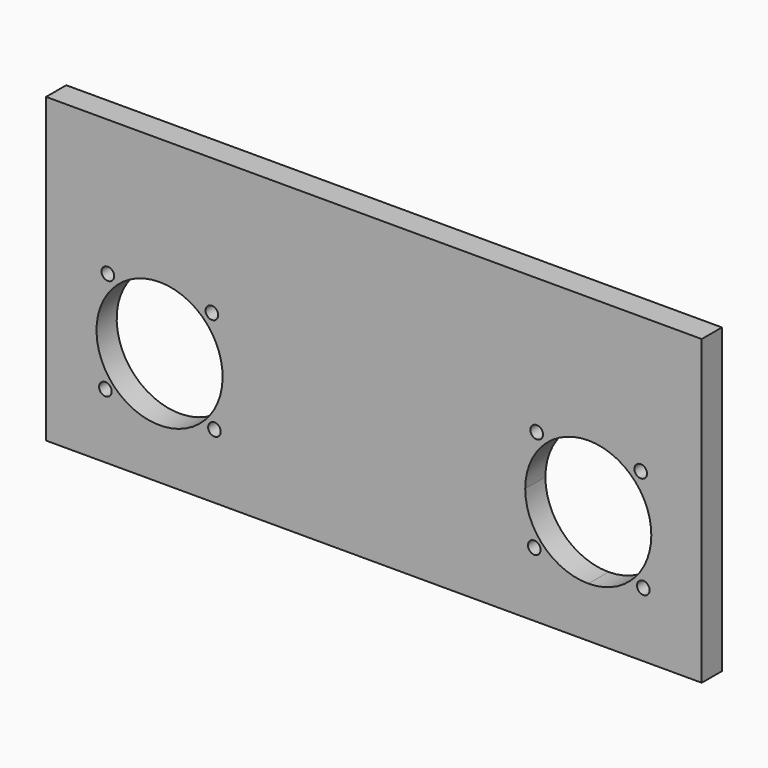
from build123d import *

# Parameters (mm, degrees)
F0_W     = 330.2
F0_H     = 152.4
F1_DEPTH = 12.7
F2_R     = 3.175
F3_DEPTH = 25.4


with BuildPart() as f1:
    # F0 (on Front) → F1 (new body)
    with BuildSketch(Plane.XZ):
        with Locations((5.4142102599, -16.3802644663)):
            Rectangle(F0_W, F0_H)
    extrude(amount=F1_DEPTH)

    # F2 (on face) → F3 (cut)
    with BuildSketch(Plane.XZ.offset(12.7)):
        with BuildLine():
            ThreePointArc((-70.7857897401, -35.4302644663), (-80.0851494374, -12.9796241636), (-102.5357897401, -3.6802644663))
            ThreePointArc((-102.5357897401, -3.6802644663), (-124.9864300428, -12.9796241636), (-134.2857897401, -35.4302644663))
            ThreePointArc((-134.2857897401, -35.4302644663), (-124.9864300428, -57.8809047689), (-102.5357897401, -67.1802644663))
            ThreePointArc((-102.5357897401, -67.1802644663), (-80.0851494374, -57.8809047689), (-70.7857897401, -35.4302644663))
        make_face()
        with BuildLine():
            ThreePointArc((81.6142102599, -35.4302644663), (90.9135700285, -57.8809048401), (113.3642104613, -67.1802644663))
            ThreePointArc((113.3642104613, -67.1802644663), (135.8148506338, -57.8809046977), (145.1142102599, -35.4302644663))
            ThreePointArc((145.1142102599, -35.4302644663), (135.8453787023, -13.0101938717), (113.4506155848, -3.6803820394))
            ThreePointArc((113.4506155848, -3.6803820394), (113.4074129624, -3.6802938596), (113.3642102599, -3.6802644663))
            ThreePointArc((113.3642102599, -3.6802644663), (90.9135699572, -12.9796241636), (81.6142102599, -35.4302644663))
        make_face()
        with Locations((-76.1955228105, -8.7878816322)):
            Circle(F2_R)
        with Locations((-128.5817733597, -8.500114777)):
            Circle(F2_R)
        with Locations((-129.8018724208, -60.0706152875)):
            Circle(F2_R)
        with Locations((-74.9057844611, -60.0706152875)):
            Circle(F2_R)
        with Locations((87.4046319652, -8.500114777)):
            Circle(F2_R)
        with Locations((139.7908825145, -8.7878816322)):
            Circle(F2_R)
        with Locations((141.0806208638, -60.0706152875)):
            Circle(F2_R)
        with Locations((86.1845329041, -60.0706152875)):
            Circle(F2_R)
    extrude(amount=-F3_DEPTH, mode=Mode.SUBTRACT)


solid = f1.part
